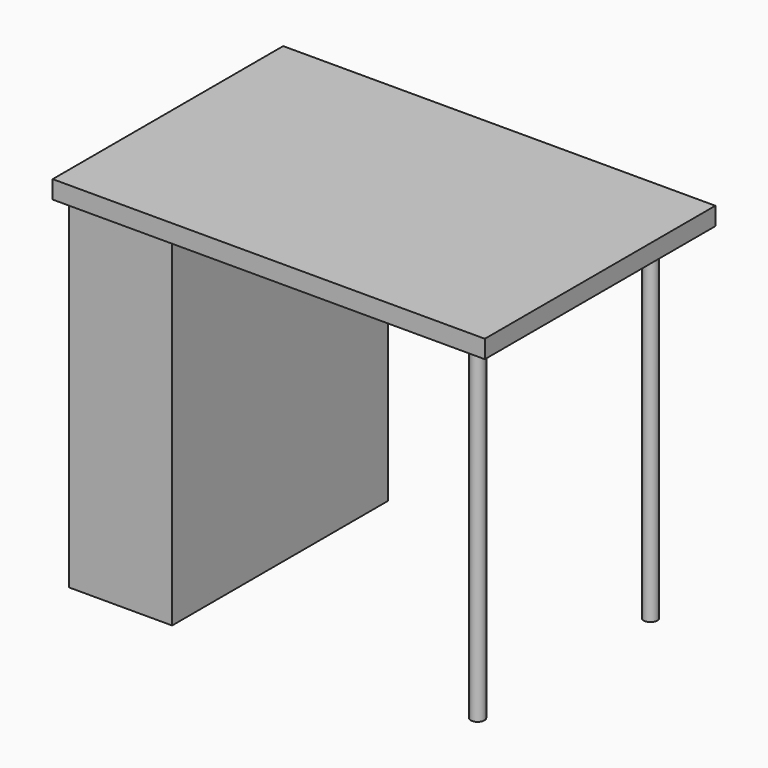
from build123d import *

# Parameters (mm, degrees)
F0_W      = 291.2060667798
F0_H      = 762
F1_DEPTH  = 25.4
F2_W      = 265.8060667798
F2_H      = 25.4
F3_DEPTH  = 914.4
F5_W      = 265.8060667798
F5_H      = 711.2
F6_DEPTH  = 25.4
F8_W      = 1219.2
F8_H      = 812.8
F8_W_2    = 291.2060667798
F8_H_2    = 762
F9_DEPTH  = 50.8
F10_R     = 50.8
F11_DEPTH = 25.4
F12_R     = 19.05
F13_DEPTH = 939.8
F17_W     = 711.2
F17_H     = 25.4
F18_DEPTH = 254


# Not quite as in the source:
# - a feature names something its author has since deleted; it is built from what else it names


with BuildPart() as f1:
    # F0 (on Top) → F1 (new body)
    with BuildSketch(Plane.XY):
        with Locations((-559.3024502769, 0)):
            Rectangle(F0_W, F0_H)
    extrude(amount=F1_DEPTH)

    # F2 (on face) → F3 (join)
    with BuildSketch(Plane.XY.offset(25.4)):
        Polygon((-413.699416887, -381), (-413.699416887, 381), (-439.099416887, 381), (-439.099416887, 355.6), (-439.099416887, -355.6), (-439.099416887, -381), align=None)
        with Locations((-572.0024502769, 368.3)):
            Rectangle(F2_W, F2_H)
        with Locations((-572.0024502769, -368.3)):
            Rectangle(F2_W, F2_H)
    extrude(amount=F3_DEPTH)

    # F5 (on offset) → F6 (join)
    with BuildSketch(Plane.XY.offset(939.8)):
        with Locations((-572.0024502769, 0)):
            Rectangle(F5_W, F5_H)
        Polygon((-413.699416887, 381), (-704.9054836667, 381), (-704.9054836667, 355.6), (-439.099416887, 355.6), (-439.099416887, -355.6), (-704.9054836667, -355.6), (-704.9054836667, -381), (-413.699416887, -381), align=None)
    extrude(amount=F6_DEPTH)

    # F17 (on face) → F18 (join)
    with BuildSketch(Plane(origin=(-439.099416887, 0, 0), x_dir=(0, -1, 0), z_dir=(-1, 0, 0))):
        with Locations((0, 520.7)):
            Rectangle(F17_W, F17_H)
    extrude(amount=F18_DEPTH)


with BuildPart() as f9:
    # F8 (on offset) → F9 (new body)
    with BuildSketch(Plane.XY.offset(965.2)):
        with Locations((-120.7054836667, 0)):
            Rectangle(F8_W, F8_H)
        with Locations((-559.3024502769, 0)):
            Rectangle(F8_W_2, F8_H_2, mode=Mode.SUBTRACT)
        with Locations((-559.3024502769, 0)):
            Rectangle(F8_W_2, F8_H_2)
    extrude(amount=F9_DEPTH)

    # F10 (on face) → F11 (join)
    with BuildSketch(Plane(origin=(0, 0, 965.2), x_dir=(1, 0, 0), z_dir=(0, 0, -1))):
        with Locations((387.2945163333, 304.8)):
            Circle(F10_R)
    extrude(amount=F11_DEPTH)

    # F12 (on face) → F13 (join)
    with BuildSketch(Plane(origin=(0, 0, 939.8), x_dir=(1, 0, 0), z_dir=(0, 0, -1))):
        with Locations((387.2945163333, 304.8)):
            Circle(F12_R)
    extrude(amount=F13_DEPTH)

    # F16: F9 across plane


with BuildPart() as f9_1:
    add(f9.part)
    add(f9.part.mirror(Plane(origin=(0, 0, 0), x_dir=(-1, 0, 0), z_dir=(0, 1, 0))))


solid = Compound([f1.part, f9_1.part])
